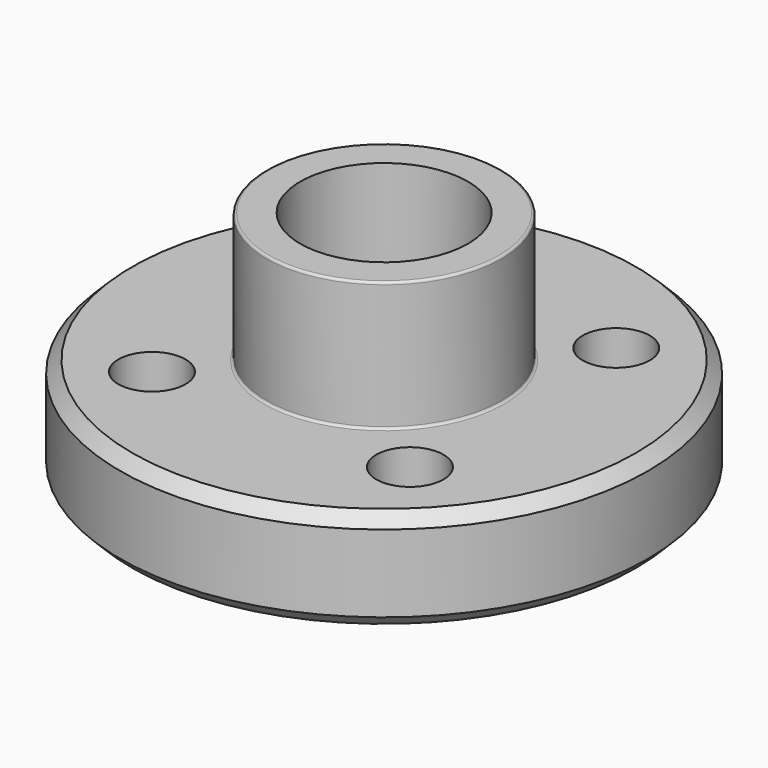
from build123d import *

# Parameters (mm, degrees)
F0_R          = 11
F0_R_2        = 1.4
F0_R_3        = 4.9
F0_R_4        = 3.5
F1_DEPTH      = 4.22
F2_DEPTH      = 5.4
F2_DEPTH_BACK = 6
F3_SIZE       = 0.5
F4_R          = 0.1


with BuildPart() as f1:
    # F0 (on Top) → F1 (new body)
    with BuildSketch(Plane.XY):
        Circle(F0_R)
        with Locations((-5.374011537, -5.374011537)):
            Circle(F0_R_2, mode=Mode.SUBTRACT)
        with Locations((5.374011537, -5.374011537)):
            Circle(F0_R_2, mode=Mode.SUBTRACT)
        with Locations((-5.374011537, 5.374011537)):
            Circle(F0_R_2, mode=Mode.SUBTRACT)
        Circle(F0_R_3, mode=Mode.SUBTRACT)
        with Locations((5.374011537, 5.374011537)):
            Circle(F0_R_2, mode=Mode.SUBTRACT)
        Circle(F0_R_3)
        Circle(F0_R_4, mode=Mode.SUBTRACT)
    extrude(amount=-F1_DEPTH)

    # F0 (on Top) → F2 (join, two sides)
    with BuildSketch(Plane.XY) as f2_sk:
        Circle(F0_R_3)
        Circle(F0_R_4, mode=Mode.SUBTRACT)
    extrude(amount=F2_DEPTH)
    extrude(f2_sk.sketch, amount=-F2_DEPTH_BACK)

    # F3
    f3_edges = [f1.edges().sort_by_distance(p)[0] for p in [
        (-11, 0, 0),
        (-11, 0, -4.22),
    ]]
    chamfer(f3_edges, length=F3_SIZE)

    # F4
    f4_edges = [f1.edges().sort_by_distance(p)[0] for p in [
        (-4.9, 0, 5.4),
        (-4.9, 0, 0),
        (-4.9, 0, -4.22),
        (-4.9, 0, -6),
    ]]
    fillet(f4_edges, radius=F4_R)


solid = f1.part
